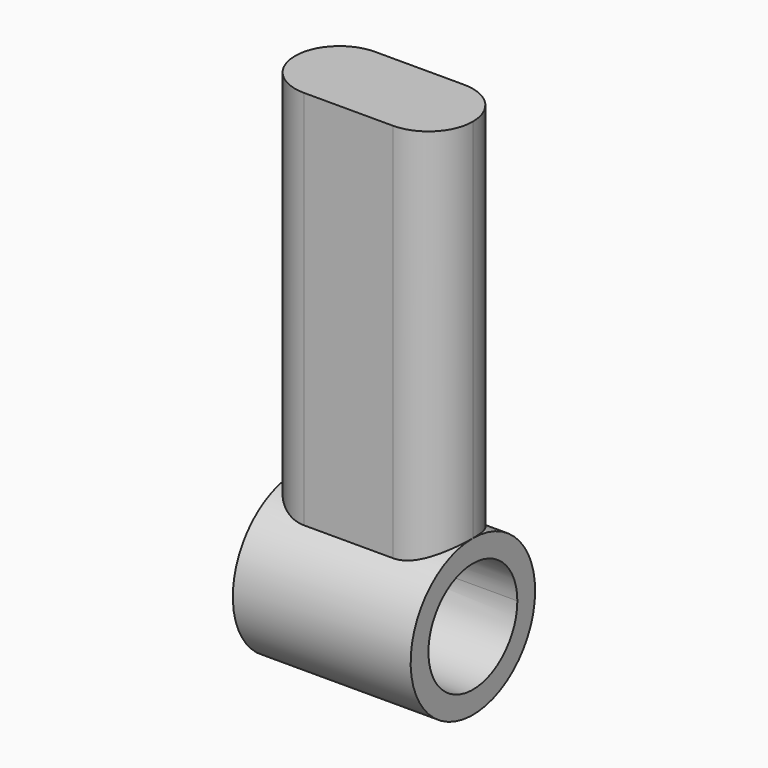
from build123d import *
from build123d import SkipClean  # not in build123d's __all__

# Parameters (mm, degrees)
F0_R     = 22.225
F0_R_2   = 15.875
F1_DEPTH = 50.8
F2_R     = 3.175
F3_DEPTH = 37.592
F5_DEPTH = 127
F6_R     = 15.875
F7_DEPTH = 70.104


with BuildPart() as f1:
    # F0 (on Right) → F1 (new body)
    with BuildSketch(Plane.YZ):
        Circle(F0_R)
        Circle(F0_R_2, mode=Mode.SUBTRACT)
    extrude(amount=F1_DEPTH)

    # F2 (on Front) → F3 (cut)
    with BuildSketch(Plane.XZ):
        with Locations((25.4, 0)):
            Circle(F2_R)
    extrude(amount=-F3_DEPTH, mode=Mode.SUBTRACT)

    # F4 (on Top) → F5 (join)
    with BuildSketch(Plane.XY):
        with BuildLine():
            ThreePointArc((12.7, 12.7), (3.7197438789, 8.9802561211), (0, 0))
            Line((0, 0), (12.7, 0))
            Line((12.7, 0), (12.7, 12.7))
        make_face()
        with BuildLine():
            Line((12.7, 0), (0, 0))
            ThreePointArc((0, 0), (3.7197438789, -8.9802561211), (12.7, -12.7))
            Line((12.7, -12.7), (12.7, 0))
        make_face()
        with BuildLine():
            Line((12.7, 12.7), (12.7, 0))
            Line((12.7, 0), (25.4, 0))
            ThreePointArc((25.4, 0), (21.6802561211, 8.9802561211), (12.7, 12.7))
        make_face()
        with BuildLine():
            Line((25.4, 0), (12.7, 0))
            Line((12.7, 0), (12.7, -12.7))
            ThreePointArc((12.7, -12.7), (21.6802561211, -8.9802561211), (25.4, 0))
        make_face()
        with BuildLine():
            Line((38.1, 12.7), (12.7, 12.7))
            ThreePointArc((12.7, 12.7), (21.6802561211, 8.9802561211), (25.4, 0))
            ThreePointArc((25.4, 0), (29.1197438789, 8.9802561211), (38.1, 12.7))
        make_face()
        with BuildLine():
            ThreePointArc((25.4, 0), (21.6802561211, -8.9802561211), (12.7, -12.7))
            Line((12.7, -12.7), (38.1, -12.7))
            ThreePointArc((38.1, -12.7), (29.1197438789, -8.9802561211), (25.4, 0))
        make_face()
        with BuildLine():
            ThreePointArc((38.1, 12.7), (29.1197438789, 8.9802561211), (25.4, 0))
            Line((25.4, 0), (38.1, 0))
            Line((38.1, 0), (38.1, 12.7))
        make_face()
        with BuildLine():
            Line((38.1, 0), (25.4, 0))
            ThreePointArc((25.4, 0), (29.1197438789, -8.9802561211), (38.1, -12.7))
            Line((38.1, -12.7), (38.1, 0))
        make_face()
        with BuildLine():
            ThreePointArc((50.8, 0), (47.0802561211, 8.9802561211), (38.1, 12.7))
            Line((38.1, 12.7), (38.1, 0))
            Line((38.1, 0), (38.1, -12.7))
            ThreePointArc((38.1, -12.7), (47.0802561211, -8.9802561211), (50.8, 0))
        make_face()
    with SkipClean():  # cleaning this boolean's faces spoils the solid; the shape is the same uncleaned
        extrude(amount=F5_DEPTH)

    # F6 (on face) → F7 (cut)
    with BuildSketch(Plane.YZ.offset(50.8)):
        Circle(F6_R)
    with SkipClean():  # cleaning this boolean's faces spoils the solid; the shape is the same uncleaned
        extrude(amount=-F7_DEPTH, mode=Mode.SUBTRACT)


solid = f1.part
